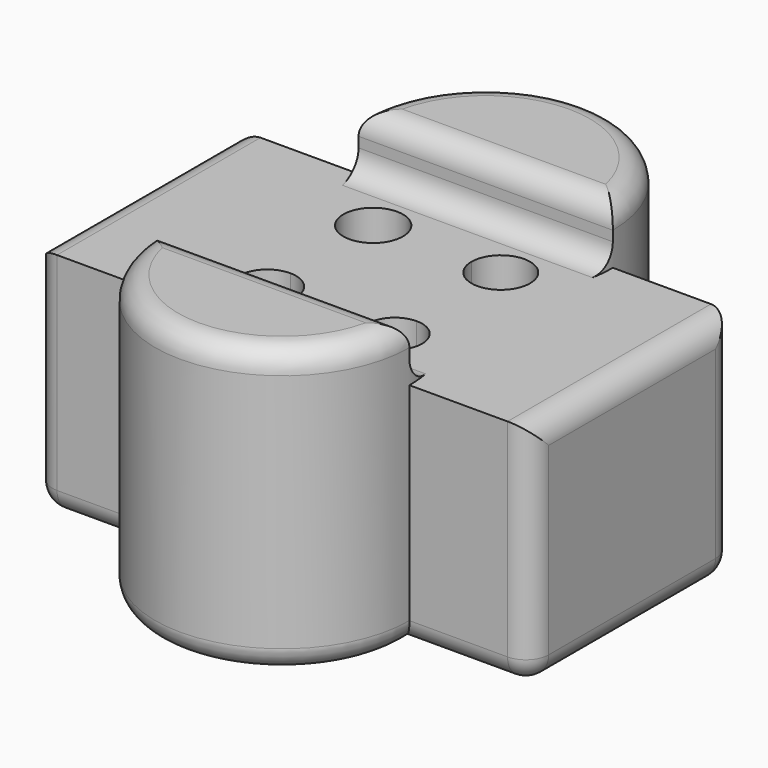
from build123d import *

# Parameters (mm, degrees)
F1_DEPTH = 51.0794
F2_DEPTH = 63.5
F3_R     = 5.08


with BuildPart() as f1:
    # F0 (on Top) → F1 (new body)
    with BuildSketch(Plane.XY):
        with BuildLine():
            ThreePointArc((-14.1626298428, 3.8117302825), (-24.4520879277, 14.1355315273), (-28.2167619251, 28.2167619251))
            Line((-28.2167619251, 28.2167619251), (-55.0714641052, 28.2167619251))
            Line((-55.0714641052, 28.2167619251), (-55.0714641052, -28.2167619251))
            Line((-55.0714641052, -28.2167619251), (-28.2167619251, -28.2167619251))
            ThreePointArc((-28.2167619251, -28.2167619251), (-24.4520879277, -14.1355315273), (-14.1626298428, -3.8117302825))
            Line((-14.1626298428, -3.8117302825), (-14.1626298428, 3.8117302825))
        make_face()
        with BuildLine():
            Line((-28.2167619251, -28.2167619251), (28.2167619251, -28.2167619251))
            ThreePointArc((28.2167619251, -28.2167619251), (24.4520879277, -14.1355315273), (14.1626298428, -3.8117302825))
            Line((14.1626298428, -3.8117302825), (14.1626298428, -8.6510551789))
            ThreePointArc((14.1626298428, -8.6510551789), (18.4362835565, -10.421260508), (20.2064888856, -14.6949142218))
            ThreePointArc((20.2064888856, -14.6949142218), (14.1626298428, -20.7387732646), (8.1187707999, -14.6949142218))
            Line((8.1187707999, -14.6949142218), (-7.75476352, -14.6949142218))
            ThreePointArc((-7.75476352, -14.6949142218), (-18.6936755725, -19.2259599515), (-14.1626298428, -8.287047899))
            Line((-14.1626298428, -8.287047899), (-14.1626298428, -3.8117302825))
            ThreePointArc((-14.1626298428, -3.8117302825), (-24.4520879277, -14.1355315273), (-28.2167619251, -28.2167619251))
        make_face()
        with BuildLine():
            ThreePointArc((14.1626298428, 3.8117302825), (24.4520879277, 14.1355315273), (28.2167619251, 28.2167619251))
            Line((28.2167619251, 28.2167619251), (-28.2167619251, 28.2167619251))
            ThreePointArc((-28.2167619251, 28.2167619251), (-24.4520879277, 14.1355315273), (-14.1626298428, 3.8117302825))
            Line((-14.1626298428, 3.8117302825), (-14.1626298428, 8.0735357175))
            ThreePointArc((-14.1626298428, 8.0735357175), (-18.8446514839, 19.3769358629), (-7.5412513385, 14.6949142218))
            Line((-7.5412513385, 14.6949142218), (7.6625943184, 14.6949142218))
            ThreePointArc((7.6625943184, 14.6949142218), (14.1626298428, 21.1949497461), (20.6626653671, 14.6949142218))
            ThreePointArc((20.6626653671, 14.6949142218), (18.75884904, 10.0986950245), (14.1626298428, 8.1948786974))
            Line((14.1626298428, 8.1948786974), (14.1626298428, 3.8117302825))
        make_face()
        with BuildLine():
            Line((55.0714641052, -28.2167619251), (55.0714641052, 28.2167619251))
            Line((55.0714641052, 28.2167619251), (28.2167619251, 28.2167619251))
            ThreePointArc((28.2167619251, 28.2167619251), (24.4520879277, 14.1355315273), (14.1626298428, 3.8117302825))
            Line((14.1626298428, 3.8117302825), (14.1626298428, -3.8117302825))
            ThreePointArc((14.1626298428, -3.8117302825), (24.4520879277, -14.1355315273), (28.2167619251, -28.2167619251))
            Line((28.2167619251, -28.2167619251), (55.0714641052, -28.2167619251))
        make_face()
        with BuildLine():
            ThreePointArc((-1.8e-09, 0), (-7.3333036869, 0.9695912358), (-14.1626298428, 3.8117302825))
            Line((-14.1626298428, 3.8117302825), (-14.1626298428, -3.8117302825))
            ThreePointArc((-14.1626298428, -3.8117302825), (-7.3333036869, -0.9695912358), (-1.8e-09, 0))
        make_face()
        with BuildLine():
            Line((14.1626298428, -3.8117302825), (14.1626298428, 3.8117302825))
            ThreePointArc((14.1626298428, 3.8117302825), (7.3333036852, 0.9695912353), (-1.8e-09, 0))
            ThreePointArc((-1.8e-09, 0), (7.3333036852, -0.9695912353), (14.1626298428, -3.8117302825))
        make_face()
        with BuildLine():
            ThreePointArc((-1.8e-09, 0), (7.3333036852, 0.9695912353), (14.1626298428, 3.8117302825))
            Line((14.1626298428, 3.8117302825), (14.1626298428, 8.1948786974))
            ThreePointArc((14.1626298428, 8.1948786974), (9.5664106455, 10.0986950245), (7.6625943184, 14.6949142218))
            Line((7.6625943184, 14.6949142218), (-7.5412513385, 14.6949142218))
            ThreePointArc((-7.5412513385, 14.6949142218), (-9.4806082016, 10.0128925806), (-14.1626298428, 8.0735357175))
            Line((-14.1626298428, 8.0735357175), (-14.1626298428, 3.8117302825))
            ThreePointArc((-14.1626298428, 3.8117302825), (-7.3333036869, 0.9695912358), (-1.8e-09, 0))
        make_face()
        with BuildLine():
            ThreePointArc((14.1626298428, -3.8117302825), (7.3333036852, -0.9695912353), (-1.8e-09, 0))
            ThreePointArc((-1.8e-09, 0), (-7.3333036869, -0.9695912358), (-14.1626298428, -3.8117302825))
            Line((-14.1626298428, -3.8117302825), (-14.1626298428, -8.287047899))
            ThreePointArc((-14.1626298428, -8.287047899), (-9.631584113, -10.163868492), (-7.75476352, -14.6949142218))
            Line((-7.75476352, -14.6949142218), (8.1187707999, -14.6949142218))
            ThreePointArc((8.1187707999, -14.6949142218), (9.888976129, -10.421260508), (14.1626298428, -8.6510551789))
            Line((14.1626298428, -8.6510551789), (14.1626298428, -3.8117302825))
        make_face()
    extrude(amount=F1_DEPTH)

    # F0 (on Top) → F2 (join)
    with BuildSketch(Plane.XY):
        with BuildLine():
            Line((-28.2167619251, 28.2167619251), (28.2167619251, 28.2167619251))
            ThreePointArc((28.2167619251, 28.2167619251), (0, 56.4335238502), (-28.2167619251, 28.2167619251))
        make_face()
        with BuildLine():
            ThreePointArc((-28.2167619251, -28.2167619251), (0, -56.4335238502), (28.2167619251, -28.2167619251))
            Line((28.2167619251, -28.2167619251), (-28.2167619251, -28.2167619251))
        make_face()
    extrude(amount=F2_DEPTH)

    # F3
    f3_edges = [f1.edges().sort_by_distance(p)[0] for p in [
        (-55.071464, 0, 0),
        (-41.644113, 28.216762, 0),
        (0, 56.433524, 0),
        (41.644113, 28.216762, 0),
        (55.071464, 0, 0),
        (41.644113, -28.216762, 0),
        (0, -56.433524, 0),
        (-41.644113, -28.216762, 0),
        (0, 28.216762, 51.0794),
        (0, 28.216762, 63.5),
        (0, -28.216762, 63.5),
        (0, -28.216762, 51.0794),
        (0, -56.433524, 63.5),
        (0, 56.433524, 63.5),
        (-55.071464, -28.216762, 25.5397),
        (-55.071464, 28.216762, 25.5397),
        (-55.071464, 0, 51.0794),
        (55.071464, -28.216762, 25.5397),
        (55.071464, 0, 51.0794),
        (55.071464, 28.216762, 25.5397),
    ]]
    fillet(f3_edges, radius=F3_R)


solid = f1.part
